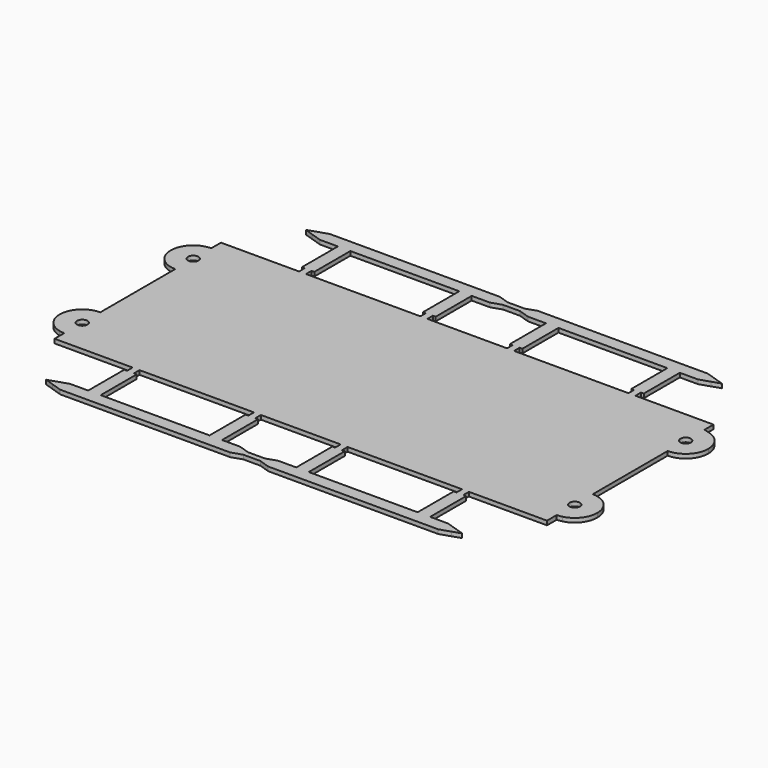
from build123d import *

# Parameters (mm, degrees)
F0_W     = 7.112
F0_H     = 2.032
F0_R     = 1.905
F0_W_2   = 2.032
F0_H_2   = 7.112
F0_W_3   = 1.524
F0_H_3   = 6.604
F0_W_4   = 6.604
F0_H_4   = 1.524
F0_W_5   = 2.54
F0_H_5   = 2.54
F1_DEPTH = 1.524


# Not quite as in the source:
# - a feature names something its author has since deleted; it is built from what else it names


with BuildPart() as f1:
    # F0 (on Top) → F1 (new body)
    with BuildSketch(Plane.XY):
        Polygon((38.1, -38.1), (38.1, 38.1), (23.495, 38.1), (20.955, 38.1), (-20.955, 38.1), (-23.495, 38.1), (-38.1, 38.1), (-38.1, -38.1), (-23.495, -38.1), (-20.955, -38.1), (20.955, -38.1), (23.495, -38.1), align=None)
        with Locations((-15.875, -30.988)):
            Rectangle(F0_W, F0_H, mode=Mode.SUBTRACT)
        with Locations((15.875, -30.988)):
            Rectangle(F0_W, F0_H, mode=Mode.SUBTRACT)
        with Locations((-25.4, -25.4)):
            Circle(F0_R, mode=Mode.SUBTRACT)
        with Locations((-30.988, -15.875)):
            Rectangle(F0_W_2, F0_H_2, mode=Mode.SUBTRACT)
        with Locations((25.4, -25.4)):
            Circle(F0_R, mode=Mode.SUBTRACT)
        with Locations((30.988, -15.875)):
            Rectangle(F0_W_2, F0_H_2, mode=Mode.SUBTRACT)
        with Locations((-30.988, 15.875)):
            Rectangle(F0_W_2, F0_H_2, mode=Mode.SUBTRACT)
        with Locations((-25.4, 25.4)):
            Circle(F0_R, mode=Mode.SUBTRACT)
        with Locations((30.988, 15.875)):
            Rectangle(F0_W_2, F0_H_2, mode=Mode.SUBTRACT)
        with Locations((25.4, 25.4)):
            Circle(F0_R, mode=Mode.SUBTRACT)
        with Locations((-15.875, 30.988)):
            Rectangle(F0_W, F0_H, mode=Mode.SUBTRACT)
        with Locations((15.875, 30.988)):
            Rectangle(F0_W, F0_H, mode=Mode.SUBTRACT)
        Polygon((52.705, 38.1), (38.1, 38.1), (38.1, -38.1), (52.705, -38.1), (55.245, -38.1), (97.155, -38.1), (99.695, -38.1), (114.3, -38.1), (114.3, 38.1), (99.695, 38.1), (97.155, 38.1), (55.245, 38.1), align=None)
        with BuildLine():
            Line((-38.1, -38.1), (-38.1, 38.1))
            Line((-38.1, 38.1), (-52.07, 33.9902844763))
            Line((-52.07, 33.9902844763), (-52.07, 33.655))
            ThreePointArc((-52.07, 33.655), (-46.2328335213, 31.2371664787), (-43.815, 25.4))
            ThreePointArc((-43.815, 25.4), (-46.2328335213, 19.5628335213), (-52.07, 17.145))
            Line((-52.07, 17.145), (-52.07, -17.145))
            ThreePointArc((-52.07, -17.145), (-46.2328335213, -19.5628335213), (-43.815, -25.4))
            ThreePointArc((-43.815, -25.4), (-46.2328335213, -31.2371664787), (-52.07, -33.655))
            Line((-52.07, -33.655), (-52.07, -33.9902844763))
            Line((-52.07, -33.9902844763), (-38.1, -38.1))
        make_face()
        with BuildLine():
            Line((128.27, 33.9902844763), (114.3, 38.1))
            Line((114.3, 38.1), (114.3, -38.1))
            Line((114.3, -38.1), (128.27, -33.9902844763))
            Line((128.27, -33.9902844763), (128.27, -33.655))
            ThreePointArc((128.27, -33.655), (120.015, -25.4), (128.27, -17.145))
            Line((128.27, -17.145), (128.27, 17.145))
            ThreePointArc((128.27, 17.145), (120.015, 25.4), (128.27, 33.655))
            Line((128.27, 33.655), (128.27, 33.9902844763))
        make_face()
        with BuildLine():
            ThreePointArc((-52.07, 33.655), (-53.0091520884, 33.6014034381), (-53.9361090652, 33.4413097165))
            ThreePointArc((-53.9361090652, 33.4413097165), (-60.2714034381, 24.4608479116), (-52.07, 17.145))
            ThreePointArc((-52.07, 17.145), (-46.2328335213, 19.5628335213), (-43.815, 25.4))
            ThreePointArc((-43.815, 25.4), (-46.2328335213, 31.2371664787), (-52.07, 33.655))
        make_face()
        with Locations((-52.07, 25.4)):
            Circle(F0_R, mode=Mode.SUBTRACT)
        with BuildLine():
            ThreePointArc((-52.07, -17.145), (-60.2714034381, -24.4608479116), (-53.9361090652, -33.4413097165))
            ThreePointArc((-53.9361090652, -33.4413097165), (-53.0091520884, -33.6014034381), (-52.07, -33.655))
            ThreePointArc((-52.07, -33.655), (-46.2328335213, -31.2371664787), (-43.815, -25.4))
            ThreePointArc((-43.815, -25.4), (-46.2328335213, -19.5628335213), (-52.07, -17.145))
        make_face()
        with Locations((-52.07, -25.4)):
            Circle(F0_R, mode=Mode.SUBTRACT)
        with BuildLine():
            ThreePointArc((128.27, -33.655), (129.2091520884, -33.6014034381), (130.1361090652, -33.4413097165))
            ThreePointArc((130.1361090652, -33.4413097165), (134.7333487966, -30.5351871761), (136.525, -25.4))
            ThreePointArc((136.525, -25.4), (134.1071664787, -19.5628335213), (128.27, -17.145))
            ThreePointArc((128.27, -17.145), (120.015, -25.4), (128.27, -33.655))
        make_face()
        with Locations((128.27, -25.4)):
            Circle(F0_R, mode=Mode.SUBTRACT)
        with BuildLine():
            ThreePointArc((136.525, 25.4), (134.7333487966, 30.5351871761), (130.1361090652, 33.4413097165))
            ThreePointArc((130.1361090652, 33.4413097165), (129.2091520884, 33.6014034381), (128.27, 33.655))
            ThreePointArc((128.27, 33.655), (120.015, 25.4), (128.27, 17.145))
            ThreePointArc((128.27, 17.145), (134.1071664787, 19.5628335213), (136.525, 25.4))
        make_face()
        with Locations((128.27, 25.4)):
            Circle(F0_R, mode=Mode.SUBTRACT)
        Polygon((-34.9994692405, 58.42), (34.9994692405, 58.42), (38.1, 59.436), (34.9994692405, 60.452), (-34.9994692405, 60.452), (-38.1, 59.436), align=None)
        Polygon((38.1, 59.436), (41.2005307595, 58.42), (111.1994692405, 58.42), (114.3, 59.436), (111.1994692405, 60.452), (41.2005307595, 60.452), align=None)
        Polygon((45.0761942089, 57.15), (51.689, 57.15), (56.261, 57.15), (76.2, 57.15), (96.139, 57.15), (100.711, 57.15), (107.3238057911, 57.15), (111.1994692405, 58.42), (41.2005307595, 58.42), align=None)
        Polygon((19.939, 57.15), (24.511, 57.15), (31.1238057911, 57.15), (34.9994692405, 58.42), (-34.9994692405, 58.42), (-31.1238057911, 57.15), (-24.511, 57.15), (-19.939, 57.15), (0, 57.15), align=None)
        Polygon((45.0761942089, 61.722), (41.2005307595, 60.452), (111.1994692405, 60.452), (107.3238057911, 61.722), (76.2, 61.722), align=None)
        Polygon((-34.9994692405, 60.452), (34.9994692405, 60.452), (31.1238057911, 61.722), (0, 61.722), (-31.1238057911, 61.722), align=None)
        Polygon((111.1994692405, -60.452), (41.2005307595, -60.452), (45.0761942089, -61.722), (76.2, -61.722), (107.3238057911, -61.722), align=None)
        Polygon((56.261, -57.15), (51.689, -57.15), (45.0761942089, -57.15), (41.2005307595, -58.42), (111.1994692405, -58.42), (107.3238057911, -57.15), (100.711, -57.15), (96.139, -57.15), (76.2, -57.15), align=None)
        Polygon((31.1238057911, -57.15), (24.511, -57.15), (19.939, -57.15), (0, -57.15), (-19.939, -57.15), (-24.511, -57.15), (-31.1238057911, -57.15), (-34.9994692405, -58.42), (34.9994692405, -58.42), align=None)
        Polygon((31.1238057911, -61.722), (34.9994692405, -60.452), (-34.9994692405, -60.452), (-31.1238057911, -61.722), (0, -61.722), align=None)
        Polygon((-23.495, 40.64), (-20.955, 40.64), (-19.939, 40.64), (-19.939, 57.15), (-24.511, 57.15), (-24.511, 40.64), align=None)
        Polygon((20.955, 40.64), (23.495, 40.64), (24.511, 40.64), (24.511, 57.15), (19.939, 57.15), (19.939, 40.64), align=None)
        Polygon((51.689, 40.64), (52.705, 40.64), (55.245, 40.64), (56.261, 40.64), (56.261, 57.15), (51.689, 57.15), align=None)
        Polygon((96.139, 40.64), (97.155, 40.64), (99.695, 40.64), (100.711, 40.64), (100.711, 57.15), (96.139, 57.15), align=None)
        Polygon((99.695, -40.64), (97.155, -40.64), (96.139, -40.64), (96.139, -57.15), (100.711, -57.15), (100.711, -40.64), align=None)
        Polygon((55.245, -40.64), (52.705, -40.64), (51.689, -40.64), (51.689, -57.15), (56.261, -57.15), (56.261, -40.64), align=None)
        Polygon((24.511, -40.64), (23.495, -40.64), (20.955, -40.64), (19.939, -40.64), (19.939, -57.15), (24.511, -57.15), align=None)
        Polygon((-19.939, -40.64), (-20.955, -40.64), (-23.495, -40.64), (-24.511, -40.64), (-24.511, -57.15), (-19.939, -57.15), align=None)
        Polygon((111.1994692405, -58.42), (41.2005307595, -58.42), (38.1, -59.436), (114.3, -59.436), align=None)
        Polygon((114.3, -59.436), (38.1, -59.436), (41.2005307595, -60.452), (111.1994692405, -60.452), align=None)
        Polygon((38.1, -59.436), (34.9994692405, -58.42), (-34.9994692405, -58.42), (-38.1, -59.436), align=None)
        Polygon((34.9994692405, -60.452), (38.1, -59.436), (-38.1, -59.436), (-34.9994692405, -60.452), align=None)
        Polygon((128.27, 38.1), (114.3, 38.1), (128.27, 33.9902844763), align=None)
        Polygon((128.27, -33.9902844763), (114.3, -38.1), (128.27, -38.1), align=None)
        Polygon((-52.07, 33.9902844763), (-38.1, 38.1), (-52.07, 38.1), align=None)
        Polygon((-52.07, -38.1), (-38.1, -38.1), (-52.07, -33.9902844763), align=None)
        with Locations((-30.988, -15.875)):
            Rectangle(F0_W_2, F0_H_2)
        with Locations((-30.988, -15.875)):
            Rectangle(F0_W_3, F0_H_3, mode=Mode.SUBTRACT)
        with Locations((-15.875, -30.988)):
            Rectangle(F0_W, F0_H)
        with Locations((-15.875, -30.988)):
            Rectangle(F0_W_4, F0_H_4, mode=Mode.SUBTRACT)
        with Locations((15.875, 30.988)):
            Rectangle(F0_W, F0_H)
        with Locations((15.875, -30.988)):
            Rectangle(F0_W, F0_H)
        with Locations((-15.875, 30.988)):
            Rectangle(F0_W, F0_H)
        with Locations((-30.988, 15.875)):
            Rectangle(F0_W_2, F0_H_2)
        with Locations((30.988, -15.875)):
            Rectangle(F0_W_2, F0_H_2)
        with Locations((30.988, 15.875)):
            Rectangle(F0_W_2, F0_H_2)
        with Locations((-25.4, 25.4)):
            Circle(F0_R)
        with Locations((25.4, 25.4)):
            Circle(F0_R)
        with Locations((-25.4, -25.4)):
            Circle(F0_R)
        with Locations((25.4, -25.4)):
            Circle(F0_R)
        with Locations((-15.875, -30.988)):
            Rectangle(F0_W_4, F0_H_4)
        with Locations((-30.988, -15.875)):
            Rectangle(F0_W_3, F0_H_3)
        with Locations((-22.225, 39.37)):
            Rectangle(F0_W_5, F0_H_5)
        with Locations((98.425, 39.37)):
            Rectangle(F0_W_5, F0_H_5)
        with Locations((22.225, 39.37)):
            Rectangle(F0_W_5, F0_H_5)
        with Locations((53.975, 39.37)):
            Rectangle(F0_W_5, F0_H_5)
        with Locations((98.425, -39.37)):
            Rectangle(F0_W_5, F0_H_5)
        with Locations((53.975, -39.37)):
            Rectangle(F0_W_5, F0_H_5)
        with Locations((-22.225, -39.37)):
            Rectangle(F0_W_5, F0_H_5)
        with Locations((22.225, -39.37)):
            Rectangle(F0_W_5, F0_H_5)
        Polygon((34.9994692405, 60.452), (38.1, 59.436), (41.2005307595, 60.452), (38.1, 60.452), align=None)
        Polygon((38.1, 59.436), (34.9994692405, 58.42), (38.1, 58.42), (41.2005307595, 58.42), align=None)
        Polygon((38.1, -58.42), (34.9994692405, -58.42), (38.1, -59.436), (41.2005307595, -58.42), align=None)
        Polygon((41.2005307595, -60.452), (38.1, -59.436), (34.9994692405, -60.452), (38.1, -60.452), align=None)
        with BuildLine():
            Line((130.1361090652, 33.4413097165), (128.27, 33.9902844763))
            Line((128.27, 33.9902844763), (128.27, 33.655))
            ThreePointArc((128.27, 33.655), (129.2091520884, 33.6014034381), (130.1361090652, 33.4413097165))
        make_face()
    extrude(amount=F1_DEPTH)


solid = f1.part
